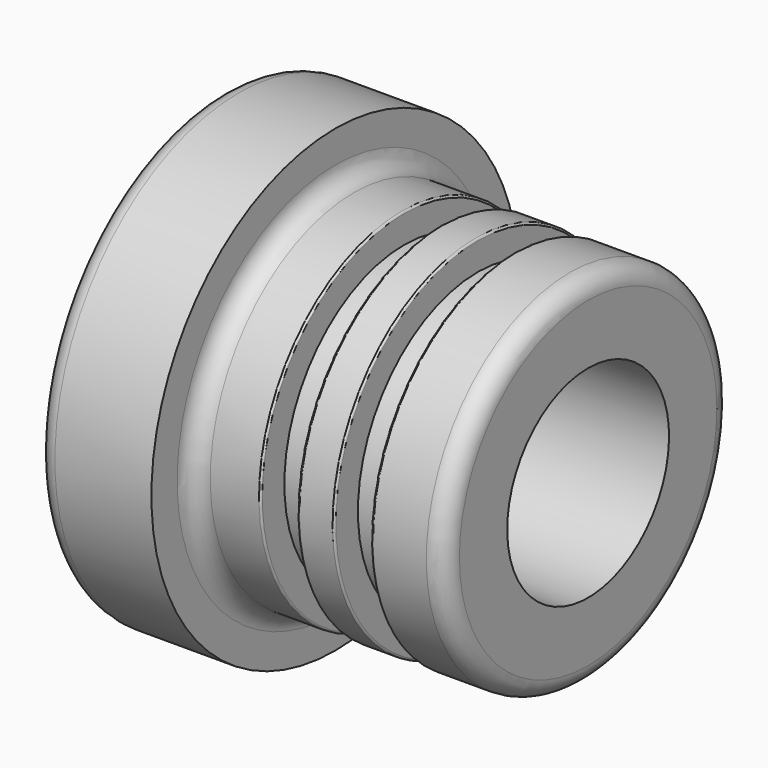
from build123d import *

# Parameters (mm, degrees)
F2_R    = 2
F3_SIZE = 1
F4_R    = 0.2


with BuildPart() as f1:
    # F0 (on Front) → F1 (revolve)
    with BuildSketch(Plane.XZ):
        Polygon((-20, 4), (-20, 2.5), (0, 2.5), (0, 11), (20, 11), (20, 19.5), (12, 19.5), (12, 16.3), (8, 16.3), (8, 19.5), (4, 19.5), (4, 16.3), (2.1880425047, 16.3), (0, 16.3), (0, 19.5), (-7.5, 19.5), (-7.5, 25), (-20, 25), (-20, 11), (-10, 11), (-10, 4), align=None)
    revolve(axis=Axis((-1.4406982809, 0, 0), (1, 0, 0)))

    # F2
    f2_edges = [f1.edges().sort_by_distance(p)[0] for p in [
        (-20, 0, -25),
        (-20, 0, -11),
        (20, 0, -19.5),
        (-7.5, 0, -19.5),
    ]]
    fillet(f2_edges, radius=F2_R)

    # F3
    f3_edges = [f1.edges().sort_by_distance(p)[0] for p in [
        (-20, 0, -4),
    ]]
    chamfer(f3_edges, length=F3_SIZE)

    # F4
    f4_edges = [f1.edges().sort_by_distance(p)[0] for p in [
        (0, 0, -19.5),
        (4, 0, -19.5),
        (8, 0, -19.5),
        (12, 0, -19.5),
    ]]
    fillet(f4_edges, radius=F4_R)


solid = f1.part
